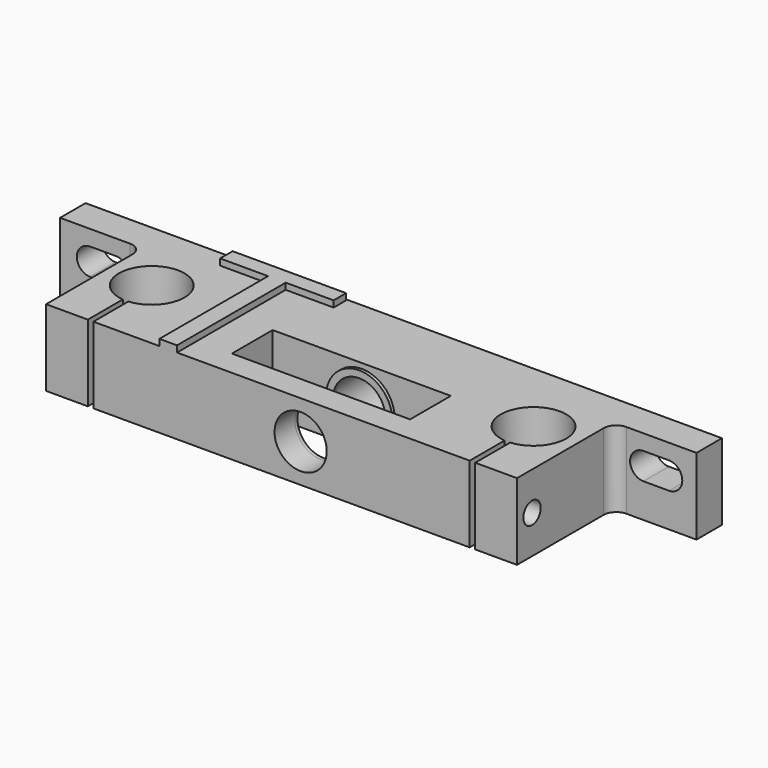
from build123d import *
from build123d import SkipClean  # not in build123d's __all__

# Parameters (mm, degrees)
F1_DEPTH      = 12
F3_DEPTH      = 12.001
F5_DEPTH      = 24.001
F6_R          = 4.1
F7_DEPTH      = 20
F8_W          = 14
F8_H          = 8
F9_DEPTH      = 12.001
F10_R         = 5.1951476321
F10_R_2       = 4.1
F11_DEPTH     = 0.5
F12_R         = 5.2529872518
F12_R_2       = 4.1
F13_DEPTH     = 0.5
F14_TEXT_SIZE = 33.3333333333
F15_DEPTH     = 1
F16_R         = 1.4
F17_DEPTH     = 18
F16_R_2       = 1.7
F18_DEPTH     = 6.5630027184
F19_R         = 2
F20_R         = 1.4
F21_DEPTH     = 18
F20_R_2       = 1.7
F22_DEPTH     = 6.5630027184
F23_R         = 2


# Not quite as in the source:
# - after a boolean that leaves OpenCascade's solid faulty, fix() repairs it
# - Text() gives the source's letters only with a copy of the font that has no kerning and outlines rounded to 1/6400 em; it was checked with that copy


with BuildPart() as f1:
    # F0 (on Top) → F1 (new body)
    with BuildSketch(Plane.XY):
        Polygon((53.6500561982, 12.3083528318), (-46.3499438018, 12.3083528318), (-46.3499438018, 7.3083528318), (-33.3499438018, 7.3083528318), (-33.3499438018, -11.6916471682), (40.6500561982, -11.6916471682), (40.6500561982, 7.3083528318), (53.6500561982, 7.3083528318), align=None)
    extrude(amount=F1_DEPTH)

    # F2 (on face) → F3 (cut, through all)
    with BuildSketch(Plane.XY.offset(12)):
        with BuildLine():
            ThreePointArc((-25.9119465202, -4.8229879659), (-22.5566480052, -3.1749512032), (-21.1999438018, 0.3083528318))
            ThreePointArc((-21.1999438018, 0.3083528318), (-29.8332478367, 4.1016486283), (-26.7879410833, -4.8229879659))
            Line((-26.7879410833, -4.8229879659), (-26.7879410833, -3.0108469723))
            Line((-26.7879410833, -3.0108469723), (-25.9119465202, -3.0108469723))
            Line((-25.9119465202, -3.0108469723), (-25.9119465202, -4.8229879659))
        make_face()
        with BuildLine():
            Line((-26.7879410833, -3.0108469723), (-26.7879410833, -4.8229879659))
            ThreePointArc((-26.7879410833, -4.8229879659), (-26.3499438018, -4.8416471682), (-25.9119465202, -4.8229879659))
            Line((-25.9119465202, -4.8229879659), (-25.9119465202, -3.0108469723))
            Line((-25.9119465202, -3.0108469723), (-26.7879410833, -3.0108469723))
        make_face()
        with BuildLine():
            ThreePointArc((-25.9119465202, -4.8229879659), (-26.3499438018, -4.8416471682), (-26.7879410833, -4.8229879659))
            Line((-26.7879410833, -4.8229879659), (-26.7879410833, -12.2696550748))
            Line((-26.7879410833, -12.2696550748), (-25.9119465202, -12.2696550748))
            Line((-25.9119465202, -12.2696550748), (-25.9119465202, -4.8229879659))
        make_face()
        with BuildLine():
            ThreePointArc((34.0880534798, -4.8229879659), (37.4433519948, -3.1749512032), (38.8000561982, 0.3083528318))
            ThreePointArc((38.8000561982, 0.3083528318), (30.1667521633, 4.1016486283), (33.2120589167, -4.8229879659))
            Line((33.2120589167, -4.8229879659), (33.2120589167, -3.0108469723))
            Line((33.2120589167, -3.0108469723), (34.0880534798, -3.0108469723))
            Line((34.0880534798, -3.0108469723), (34.0880534798, -4.8229879659))
        make_face()
        with BuildLine():
            Line((33.2120589167, -3.0108469723), (33.2120589167, -4.8229879659))
            ThreePointArc((33.2120589167, -4.8229879659), (33.6500561982, -4.8416471682), (34.0880534798, -4.8229879659))
            Line((34.0880534798, -4.8229879659), (34.0880534798, -3.0108469723))
            Line((34.0880534798, -3.0108469723), (33.2120589167, -3.0108469723))
        make_face()
        with BuildLine():
            ThreePointArc((34.0880534798, -4.8229879659), (33.6500561982, -4.8416471682), (33.2120589167, -4.8229879659))
            Line((33.2120589167, -4.8229879659), (33.2120589167, -12.2696550748))
            Line((33.2120589167, -12.2696550748), (34.0880534798, -12.2696550748))
            Line((34.0880534798, -12.2696550748), (34.0880534798, -4.8229879659))
        make_face()
    extrude(amount=-F3_DEPTH, mode=Mode.SUBTRACT)

    # F4 (on face) → F5 (cut, through all)
    with BuildSketch(Plane(origin=(0, 12.3083528318, 0), x_dir=(-1, 0, 0), z_dir=(0, 1, 0))):
        with BuildLine():
            Line((-45.3214800954, 9.5596171677), (-49.3214800954, 9.5596171677))
            ThreePointArc((-49.3214800954, 9.5596171677), (-51.4214800954, 7.4596171677), (-49.3214800954, 5.3596171677))
            Line((-49.3214800954, 5.3596171677), (-45.3214800954, 5.3596171677))
            ThreePointArc((-45.3214800954, 5.3596171677), (-43.2214800954, 7.4596171677), (-45.3214800954, 9.5596171677))
        make_face()
        with BuildLine():
            ThreePointArc((37.6219116151, 9.5596171677), (35.5219116151, 7.4596171677), (37.6219116151, 5.3596171677))
            Line((37.6219116151, 5.3596171677), (41.6219116151, 5.3596171677))
            ThreePointArc((41.6219116151, 5.3596171677), (43.7219116151, 7.4596171677), (41.6219116151, 9.5596171677))
            Line((41.6219116151, 9.5596171677), (37.6219116151, 9.5596171677))
        make_face()
    extrude(amount=-F5_DEPTH, mode=Mode.SUBTRACT)

    # F6 (on face) → F7 (cut)
    with BuildSketch(Plane.XZ.offset(11.6916471682)):
        with Locations((6.6500561982, 6)):
            Circle(F6_R)
    extrude(amount=-F7_DEPTH, mode=Mode.SUBTRACT)

    # F8 (on face) → F9 (cut, through all)
    with BuildSketch(Plane.XY.offset(12)):
        with Locations((-0.3499438018, -3.6916471682)):
            Rectangle(F8_W, F8_H)
        with Locations((13.6500561982, -3.6916471682)):
            Rectangle(F8_W, F8_H)
    extrude(amount=-F9_DEPTH, mode=Mode.SUBTRACT)

    # F10 (on face) → F11 (join)
    with BuildSketch(Plane.XZ.offset(-0.3083528318)):
        with Locations((6.6500561982, 6)):
            Circle(F10_R)
        with Locations((6.6500561982, 6)):
            Circle(F10_R_2, mode=Mode.SUBTRACT)
    extrude(amount=F11_DEPTH)

    # F12 (on face) → F13 (join)
    with BuildSketch(Plane(origin=(0, -7.6916471682, 0), x_dir=(-1, 0, 0), z_dir=(0, 1, 0))):
        with Locations((-6.6500561982, 6)):
            Circle(F12_R)
        with Locations((-6.6500561982, 6)):
            Circle(F12_R_2, mode=Mode.SUBTRACT)
    with SkipClean():  # cleaning this boolean's faces spoils the solid; the shape is the same uncleaned
        extrude(amount=F13_DEPTH)

    # F14 (on face) → F15 (join)
    with BuildSketch(Plane.XY.offset(12)):
        with Locations((-23.367214418, -11.6916471682)):
            Text('T', F14_TEXT_SIZE, font='Open Sans', text_align=(TextAlign.LEFT, TextAlign.BOTTOM))
    extrude(amount=F15_DEPTH)

    add(f1.part.fix(), mode=Mode.REPLACE)

    # F16 (on face) → F17 (cut)
    with BuildSketch(Plane.YZ.offset(40.6500561982)):
        with Locations((-8.7363375351, 6)):
            Circle(F16_R)
    extrude(amount=-F17_DEPTH, mode=Mode.SUBTRACT)

    # F16 (on face) → F18 (cut, through all)
    with BuildSketch(Plane.YZ.offset(40.6500561982)):
        with Locations((-8.7363375351, 6)):
            Circle(F16_R_2)
        with Locations((-8.7363375351, 6)):
            Circle(F16_R, mode=Mode.SUBTRACT)
        with Locations((-8.7363375351, 6)):
            Circle(F16_R)
    extrude(amount=-F18_DEPTH, mode=Mode.SUBTRACT)

    # F19
    f19_edges = [f1.edges().sort_by_distance(p)[0] for p in [
        (40.650056, 7.308353, 6),
    ]]
    fillet(f19_edges, radius=F19_R)

    # F20 (on face) → F21 (cut)
    with BuildSketch(Plane(origin=(-33.3499438018, 0, 0), x_dir=(0, -1, 0), z_dir=(-1, 0, 0))):
        with Locations((8.7602175772, 6.004051771)):
            Circle(F20_R)
    extrude(amount=-F21_DEPTH, mode=Mode.SUBTRACT)

    # F20 (on face) → F22 (cut, through all)
    with BuildSketch(Plane(origin=(-33.3499438018, 0, 0), x_dir=(0, -1, 0), z_dir=(-1, 0, 0))):
        with Locations((8.7602175772, 6.004051771)):
            Circle(F20_R_2)
        with Locations((8.7602175772, 6.004051771)):
            Circle(F20_R, mode=Mode.SUBTRACT)
        with Locations((8.7602175772, 6.004051771)):
            Circle(F20_R)
    extrude(amount=-F22_DEPTH, mode=Mode.SUBTRACT)

    # F23
    f23_edges = [f1.edges().sort_by_distance(p)[0] for p in [
        (-33.349944, 7.308353, 6),
    ]]
    fillet(f23_edges, radius=F23_R)


solid = f1.part
